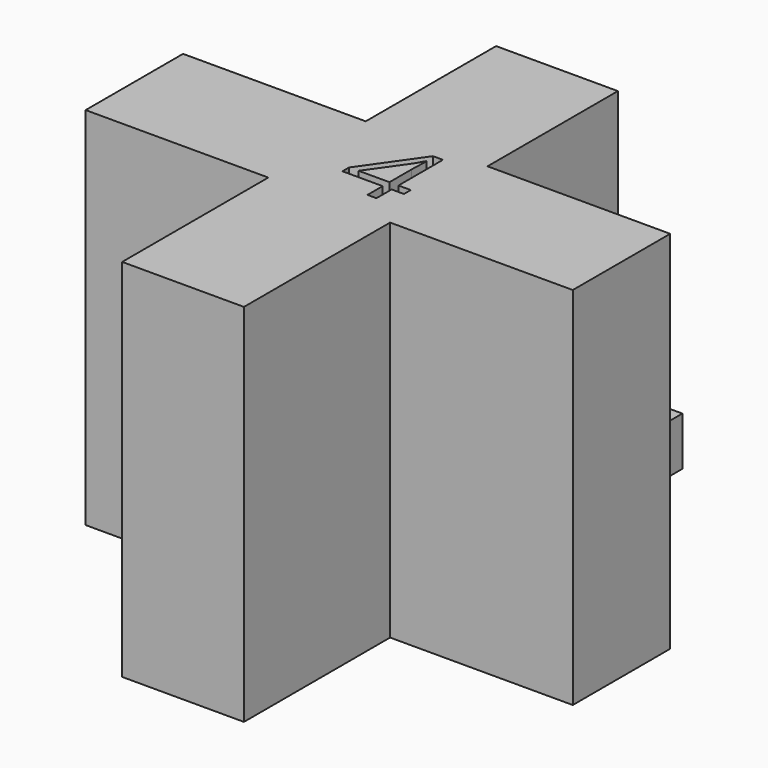
from build123d import *

# Parameters (mm, degrees)
F0_W         = 12.7
F0_H         = 57.15
F1_DEPTH     = 5.08
F2_W         = 50.8
F2_H         = 12.7
F3_DEPTH     = 38.1
F4_W         = 12.7
F4_H         = 48.7413735385
F5_DEPTH     = 33.02
F6_TEXT_SIZE = 12.0747026004
F7_DEPTH     = 2.54


# Not quite as in the source:
# - Text() gives the source's letters only with a copy of the font that has no kerning and outlines rounded to 1/6400 em; it was checked with that copy


with BuildPart() as f1:
    # F0 (on Top) → F1 (new body)
    with BuildSketch(Plane.XY):
        with Locations((-37.0165128261, 2.9978602284)):
            Rectangle(F0_W, F0_H)
    extrude(amount=F1_DEPTH)

    # F2 (on Top) → F3 (join)
    with BuildSketch(Plane.XY):
        with Locations((-37.0165128261, -0.1771397716)):
            Rectangle(F2_W, F2_H)
    extrude(amount=F3_DEPTH)

    # F4 (on face) → F5 (join)
    with BuildSketch(Plane.XY.offset(5.08)):
        with Locations((-37.0165128261, -1.2064530024)):
            Rectangle(F4_W, F4_H)
    extrude(amount=F5_DEPTH)

    # F6 (on face) → F7 (cut)
    with BuildSketch(Plane.XY.offset(38.1)):
        with Locations((-39.5974777639, -3.8714513648)):
            Text('4', F6_TEXT_SIZE, font='Open Sans', text_align=(TextAlign.LEFT, TextAlign.BOTTOM))
    extrude(amount=-F7_DEPTH, mode=Mode.SUBTRACT)


solid = f1.part
